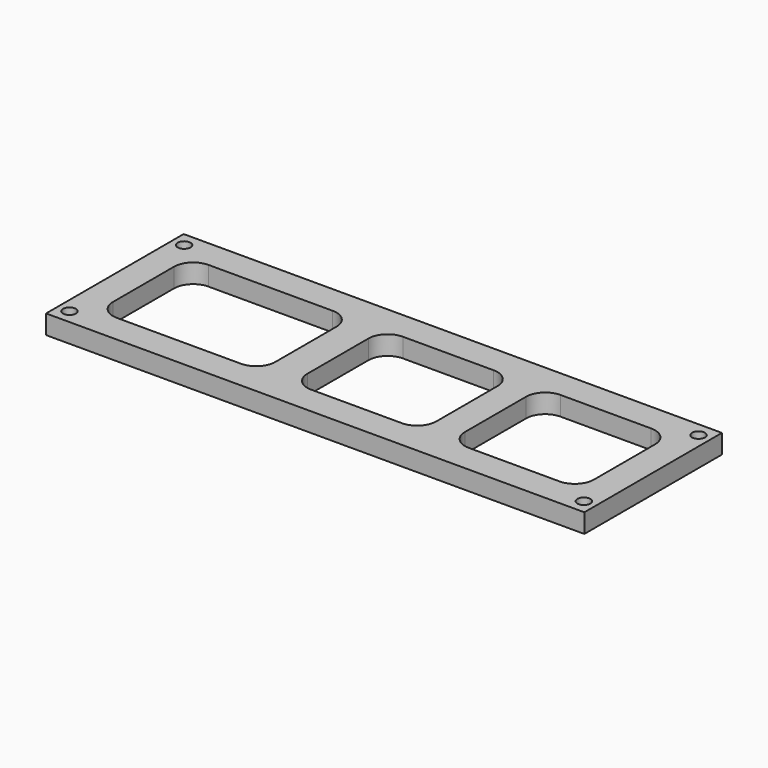
from build123d import *

# Parameters (mm, degrees)
F0_W     = 112.7
F0_H     = 36
F1_DEPTH = 4
F2_R     = 1.35
F3_DEPTH = 4.001
F4_W     = 34
F4_H     = 24
F4_W_2   = 27
F5_DEPTH = 4.001
F6_R     = 4


# Not quite as in the source:
# - a feature names something its author has since deleted; it is built from what else it names


with BuildPart() as f1:
    # F0 (on Top) → F1 (new body)
    with BuildSketch(Plane.XY):
        Rectangle(F0_W, F0_H)
    extrude(amount=F1_DEPTH)

    # F2 (on face) → F3 (cut, through all)
    with BuildSketch(Plane(origin=(0, 0, 0), x_dir=(1, 0, 0), z_dir=(0, 0, -1))):
        with Locations((-53.85, 15)):
            Circle(F2_R)
        with Locations((-53.85, -15)):
            Circle(F2_R)
        with Locations((53.85, 15)):
            Circle(F2_R)
        with Locations((53.85, -15)):
            Circle(F2_R)
    extrude(amount=-F3_DEPTH, mode=Mode.SUBTRACT)

    # F4 (on face) → F5 (cut, through all)
    with BuildSketch(Plane(origin=(0, 0, 0), x_dir=(1, 0, 0), z_dir=(0, 0, -1))):
        with Locations((-33.35, 0)):
            Rectangle(F4_W, F4_H)
        with Locations((3.85, 0)):
            Rectangle(F4_W_2, F4_H)
        with Locations((36.85, 0)):
            Rectangle(F4_W_2, F4_H)
    extrude(amount=-F5_DEPTH, mode=Mode.SUBTRACT)

    # F6
    f6_edges = [f1.edges().sort_by_distance(p)[0] for p in [
        (-16.35, -12, 2),
        (-50.35, -12, 2),
        (-50.35, 12, 2),
        (-16.35, 12, 2),
        (-9.65, -12, 2),
        (23.35, -12, 2),
        (-9.65, 12, 2),
        (17.35, -12, 2),
        (50.35, -12, 2),
        (50.35, 12, 2),
        (23.35, 12, 2),
        (17.35, 12, 2),
    ]]
    fillet(f6_edges, radius=F6_R)


solid = f1.part
